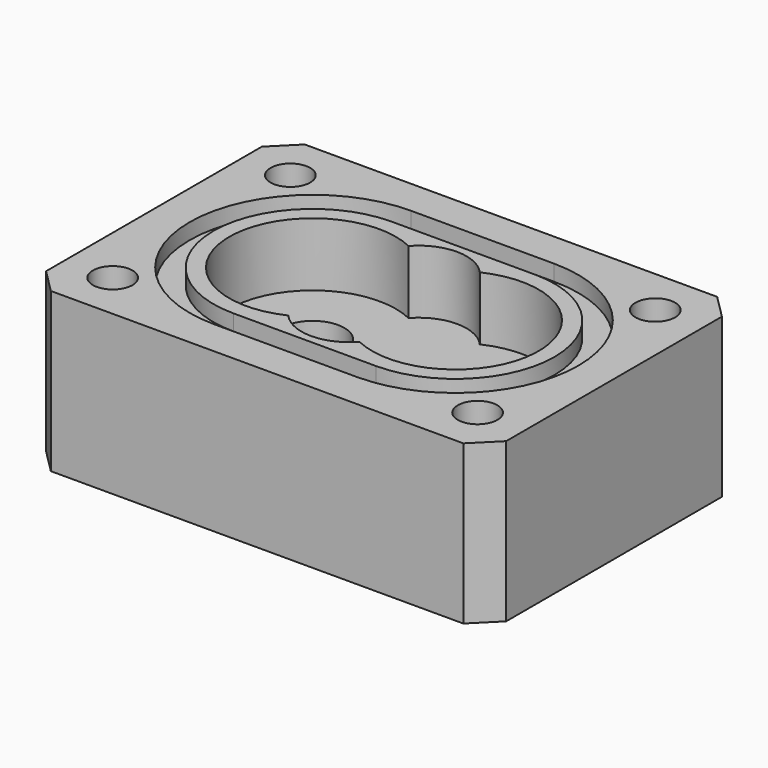
from build123d import *

# Parameters (mm, degrees)
F0_W     = 29
F0_H     = 20
F0_R     = 1.25
F0_R_2   = 2
F1_DEPTH = 10
F2_DEPTH = 5
F3_DEPTH = 1
F4_DEPTH = 8
F5_DEPTH = 4
F6_R     = 4
F6_R_2   = 2
F7_DEPTH = 1
F8_SIZE  = 1.5


# Not quite as in the source:
# - a feature names something its author has since deleted; it is built from what else it names


with BuildPart() as f1:
    # F0 (on Top) → F1 (new body)
    with BuildSketch(Plane.XY):
        with Locations((14.5, -10)):
            Rectangle(F0_W, F0_H)
        with Locations((3, -17)):
            Circle(F0_R, mode=Mode.SUBTRACT)
        with Locations((26, -17)):
            Circle(F0_R, mode=Mode.SUBTRACT)
        with Locations((3, -3)):
            Circle(F0_R, mode=Mode.SUBTRACT)
        with BuildLine():
            Line((19, -17.75), (10, -17.75))
            ThreePointArc((10, -17.75), (2.25, -10), (10, -2.25))
            Line((10, -2.25), (19, -2.25))
            ThreePointArc((19, -2.25), (26.75, -10), (19, -17.75))
        make_face(mode=Mode.SUBTRACT)
        with Locations((26, -3)):
            Circle(F0_R, mode=Mode.SUBTRACT)
        with BuildLine():
            ThreePointArc((10, -2.25), (2.25, -10), (10, -17.75))
            Line((10, -17.75), (19, -17.75))
            ThreePointArc((19, -17.75), (26.75, -10), (19, -2.25))
            Line((19, -2.25), (10, -2.25))
        make_face()
        with BuildLine():
            ThreePointArc((10, -16.25), (3.75, -10), (10, -3.75))
            Line((10, -3.75), (19, -3.75))
            ThreePointArc((19, -3.75), (25.25, -10), (19, -16.25))
            Line((19, -16.25), (10, -16.25))
        make_face(mode=Mode.SUBTRACT)
        with BuildLine():
            Line((19, -3.75), (10, -3.75))
            ThreePointArc((10, -3.75), (3.75, -10), (10, -16.25))
            Line((10, -16.25), (19, -16.25))
            ThreePointArc((19, -16.25), (25.25, -10), (19, -3.75))
        make_face()
        with BuildLine():
            ThreePointArc((16.7443308628, -5.25927677), (24.25, -10), (16.7443308628, -14.74072323))
            ThreePointArc((16.7443308628, -14.74072323), (14.5, -15.75), (12.2556691372, -14.74072323))
            ThreePointArc((12.2556691372, -14.74072323), (4.75, -10), (12.2556691372, -5.25927677))
            ThreePointArc((12.2556691372, -5.25927677), (14.5, -4.25), (16.7443308628, -5.25927677))
        make_face(mode=Mode.SUBTRACT)
        with BuildLine():
            ThreePointArc((12.2556691372, -14.74072323), (14.5, -15.75), (16.7443308628, -14.74072323))
            ThreePointArc((16.7443308628, -14.74072323), (24.25, -10), (16.7443308628, -5.25927677))
            ThreePointArc((16.7443308628, -5.25927677), (14.5, -4.25), (12.2556691372, -5.25927677))
            ThreePointArc((12.2556691372, -5.25927677), (4.75, -10), (12.2556691372, -14.74072323))
        make_face()
        with Locations((10, -10)):
            Circle(F0_R_2, mode=Mode.SUBTRACT)
        with Locations((19, -10)):
            Circle(F0_R_2, mode=Mode.SUBTRACT)
        with Locations((19, -10)):
            Circle(F0_R_2)
        with Locations((3, -17)):
            Circle(F0_R)
        with Locations((26, -3)):
            Circle(F0_R)
    extrude(amount=-F1_DEPTH)

    # F0 (on Top) → F2 (cut)
    with BuildSketch(Plane.XY):
        with Locations((3, -3)):
            Circle(F0_R)
        with Locations((26, -3)):
            Circle(F0_R)
        with Locations((26, -17)):
            Circle(F0_R)
        with Locations((3, -17)):
            Circle(F0_R)
    extrude(amount=-F2_DEPTH, mode=Mode.SUBTRACT)

    # F0 (on Top) → F3 (cut)
    with BuildSketch(Plane.XY):
        with BuildLine():
            ThreePointArc((10, -2.25), (2.25, -10), (10, -17.75))
            Line((10, -17.75), (19, -17.75))
            ThreePointArc((19, -17.75), (26.75, -10), (19, -2.25))
            Line((19, -2.25), (10, -2.25))
        make_face()
        with BuildLine():
            ThreePointArc((10, -16.25), (3.75, -10), (10, -3.75))
            Line((10, -3.75), (19, -3.75))
            ThreePointArc((19, -3.75), (25.25, -10), (19, -16.25))
            Line((19, -16.25), (10, -16.25))
        make_face(mode=Mode.SUBTRACT)
    extrude(amount=-F3_DEPTH, mode=Mode.SUBTRACT)

    # F0 (on Top) → F4 (cut)
    with BuildSketch(Plane.XY):
        with Locations((19, -10)):
            Circle(F0_R_2)
    extrude(amount=-F4_DEPTH, mode=Mode.SUBTRACT)

    # F0 (on Top) → F5 (cut)
    with BuildSketch(Plane.XY):
        with BuildLine():
            ThreePointArc((12.2556691372, -14.74072323), (14.5, -15.75), (16.7443308628, -14.74072323))
            ThreePointArc((16.7443308628, -14.74072323), (24.25, -10), (16.7443308628, -5.25927677))
            ThreePointArc((16.7443308628, -5.25927677), (14.5, -4.25), (12.2556691372, -5.25927677))
            ThreePointArc((12.2556691372, -5.25927677), (4.75, -10), (12.2556691372, -14.74072323))
        make_face()
        with Locations((10, -10)):
            Circle(F0_R_2, mode=Mode.SUBTRACT)
        with Locations((19, -10)):
            Circle(F0_R_2, mode=Mode.SUBTRACT)
    extrude(amount=-F5_DEPTH, mode=Mode.SUBTRACT)

    # F6 (on face) → F7 (cut)
    with BuildSketch(Plane(origin=(0, 0, -10), x_dir=(1, 0, 0), z_dir=(0, 0, -1))):
        with Locations((10, 10)):
            Circle(F6_R)
        with Locations((10, 10)):
            Circle(F6_R_2, mode=Mode.SUBTRACT)
    extrude(amount=-F7_DEPTH, mode=Mode.SUBTRACT)

    # F8
    f8_edges = [f1.edges().sort_by_distance(p)[0] for p in [
        (29, -20, -5),
        (0, -20, -5),
        (0, 0, -5),
        (29, 0, -5),
    ]]
    chamfer(f8_edges, length=F8_SIZE)


solid = f1.part
